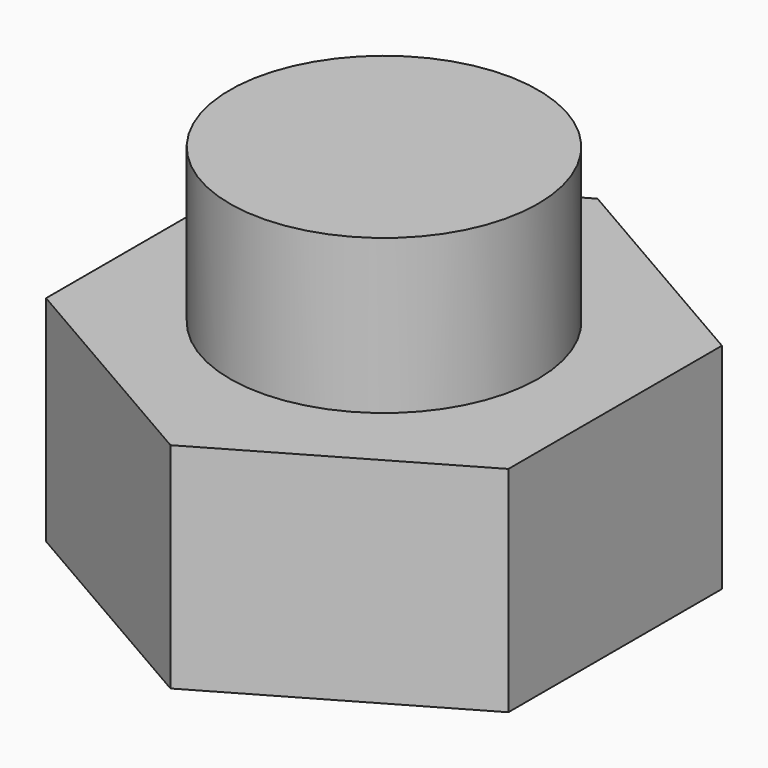
from build123d import *

# Parameters (mm, degrees)
F1_DEPTH = 13.9
F2_R     = 10
F3_DEPTH = 10


# Not quite as in the source:
# - the program builds the solid bodies; features that only make, move or delete a surface that nothing else refers to are left out


with BuildPart() as f1:
    # F0 (on Top) → F1 (new body)
    with BuildSketch(Plane.XY):
        Polygon((15, 8.6602540378), (0, 17.3205080757), (-15, 8.6602540378), (-15, -8.6602540378), (0, -17.3205080757), (15, -8.6602540378), align=None)
    extrude(amount=F1_DEPTH)

    # F2 (on face) → F3 (join)
    with BuildSketch(Plane.XY.offset(13.9)):
        Circle(F2_R)
    extrude(amount=F3_DEPTH)


solid = f1.part
